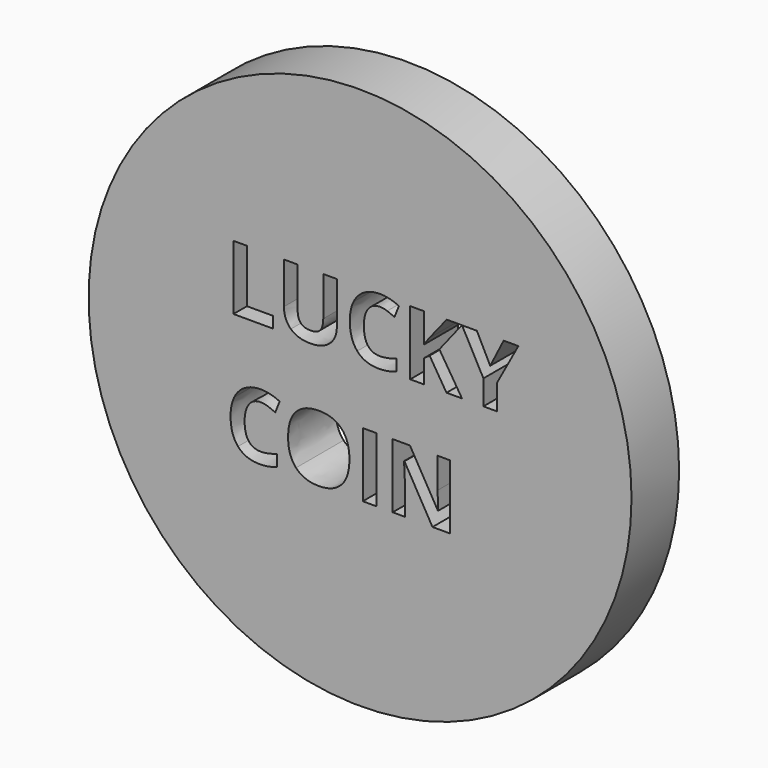
from build123d import *

# Parameters (mm, degrees)
F0_R     = 57.932951026
F0_W     = 2.9168109343
F0_H     = 13.753260226
F1_DEPTH = 12.7


with BuildPart() as f1:
    # F0 (on Front) → F1 (new body)
    with BuildSketch(Plane.XZ):
        Circle(F0_R)
        with BuildLine():
            add(Edge.make_bspline(
                [(-19.6506091277, -8.0144570558), (-20.4302314517, -7.7420407611), (-21.1827626525, -7.7420407611)],
                knots=[0, 0, 0, 1, 1, 1], degree=2))
            add(Edge.make_bspline(
                [(-21.1827626525, -7.7420407611), (-22.8293009199, -7.7420407611), (-23.7323383609, -8.9792020552)],
                knots=[0, 0, 0, 1, 1, 1], degree=2))
            add(Edge.make_bspline(
                [(-23.7323383609, -8.9792020552), (-24.6353758019, -10.2163633494), (-24.6353758019, -12.425794955)],
                knots=[0, 0, 0, 1, 1, 1], degree=2))
            add(Edge.make_bspline(
                [(-24.6353758019, -12.425794955), (-24.6353758019, -17.0252656543), (-21.1827626525, -17.0252656543)],
                knots=[0, 0, 0, 1, 1, 1], degree=2))
            add(Edge.make_bspline(
                [(-21.1827626525, -17.0252656543), (-19.7348926222, -17.0252656543), (-17.6759672568, -16.3028357015)],
                knots=[0, 0, 0, 1, 1, 1], degree=2))
            Line((-17.6759672568, -16.3028357015), (-17.6759672568, -18.7470570418))
            add(Edge.make_bspline(
                [(-17.6759672568, -18.7470570418), (-19.3676573962, -19.4544363705), (-21.4566840096, -19.4544363705)],
                knots=[0, 0, 0, 1, 1, 1], degree=2))
            add(Edge.make_bspline(
                [(-21.4566840096, -19.4544363705), (-24.4577784385, -19.4544363705), (-26.0471243346, -17.6333108646)],
                knots=[0, 0, 0, 1, 1, 1], degree=2))
            add(Edge.make_bspline(
                [(-26.0471243346, -17.6333108646), (-27.6364702307, -15.8121853586), (-27.6364702307, -12.4077342061)],
                knots=[0, 0, 0, 1, 1, 1], degree=2))
            add(Edge.make_bspline(
                [(-27.6364702307, -12.4077342061), (-27.6364702307, -10.2615152214), (-26.8553428443, -8.6480883269)],
                knots=[0, 0, 0, 1, 1, 1], degree=2))
            add(Edge.make_bspline(
                [(-26.8553428443, -8.6480883269), (-26.0742154578, -7.0346614323), (-24.6112948034, -6.175270801)],
                knots=[0, 0, 0, 1, 1, 1], degree=2))
            add(Edge.make_bspline(
                [(-24.6112948034, -6.175270801), (-23.1483741491, -5.3158801697), (-21.1827626525, -5.3158801697)],
                knots=[0, 0, 0, 1, 1, 1], degree=2))
            add(Edge.make_bspline(
                [(-21.1827626525, -5.3158801697), (-19.1810296584, -5.3158801697), (-17.1582257906, -6.2821302315)],
                knots=[0, 0, 0, 1, 1, 1], degree=2))
            Line((-17.1582257906, -6.2821302315), (-18.0973847292, -8.6541085765))
            add(Edge.make_bspline(
                [(-18.0973847292, -8.6541085765), (-18.8709868037, -8.2868733505), (-19.6506091277, -8.0144570558)],
                knots=[0, 0, 0, 1, 1, 1], degree=2))
        make_face(mode=Mode.SUBTRACT)
        with BuildLine():
            add(Edge.make_bspline(
                [(-3.9467880292, -7.1204499892), (-2.267138389, -8.9460906824), (-2.267138389, -12.3686025837)],
                knots=[0, 0, 0, 1, 1, 1], degree=2))
            add(Edge.make_bspline(
                [(-2.267138389, -12.3686025837), (-2.267138389, -15.7850942354), (-3.9603335908, -17.619765303)],
                knots=[0, 0, 0, 1, 1, 1], degree=2))
            add(Edge.make_bspline(
                [(-3.9603335908, -17.619765303), (-5.6535287926, -19.4544363705), (-8.814159836, -19.4544363705)],
                knots=[0, 0, 0, 1, 1, 1], degree=2))
            add(Edge.make_bspline(
                [(-8.814159836, -19.4544363705), (-11.9747908794, -19.4544363705), (-13.6679860812, -17.619765303)],
                knots=[0, 0, 0, 1, 1, 1], degree=2))
            add(Edge.make_bspline(
                [(-13.6679860812, -17.619765303), (-15.3611812831, -15.7850942354), (-15.3611812831, -12.3505418349)],
                knots=[0, 0, 0, 1, 1, 1], degree=2))
            add(Edge.make_bspline(
                [(-15.3611812831, -12.3505418349), (-15.3611812831, -8.9159894344), (-13.663470894, -7.1053993652)],
                knots=[0, 0, 0, 1, 1, 1], degree=2))
            add(Edge.make_bspline(
                [(-13.663470894, -7.1053993652), (-11.965760505, -5.2948092961), (-8.7960990872, -5.2948092961)],
                knots=[0, 0, 0, 1, 1, 1], degree=2))
            add(Edge.make_bspline(
                [(-8.7960990872, -5.2948092961), (-5.6264376694, -5.2948092961), (-3.9467880292, -7.1204499892)],
                knots=[0, 0, 0, 1, 1, 1], degree=2))
        make_face(mode=Mode.SUBTRACT)
        with Locations((2.0418552669, -12.3881683949)):
            Rectangle(F0_W, F0_H, mode=Mode.SUBTRACT)
        with BuildLine():
            Line((19.1619400853, -5.5115382819), (19.1619400853, -19.2647985079))
            Line((19.1619400853, -19.2647985079), (15.4564764525, -19.2647985079))
            Line((15.4564764525, -19.2647985079), (9.4723483437, -8.8618071879))
            Line((9.4723483437, -8.8618071879), (9.3880648492, -8.8618071879))
            add(Edge.make_bspline(
                [(9.3880648492, -8.8618071879), (9.5686723374, -11.6160713829), (9.5686723374, -12.793030181)],
                knots=[0, 0, 0, 1, 1, 1], degree=2))
            Line((9.5686723374, -12.793030181), (9.5686723374, -19.2647985079))
            Line((9.5686723374, -19.2647985079), (6.9619042578, -19.2647985079))
            Line((6.9619042578, -19.2647985079), (6.9619042578, -5.5115382819))
            Line((6.9619042578, -5.5115382819), (10.6402767673, -5.5115382819))
            Line((10.6402767673, -5.5115382819), (16.612364377, -15.8121853586))
            Line((16.612364377, -15.8121853586), (16.6785871226, -15.8121853586))
            add(Edge.make_bspline(
                [(16.6785871226, -15.8121853586), (16.5371112569, -13.1301641589), (16.5371112569, -12.0224382313)],
                knots=[0, 0, 0, 1, 1, 1], degree=2))
            Line((16.5371112569, -12.0224382313), (16.5371112569, -5.5115382819))
            Line((16.5371112569, -5.5115382819), (19.1619400853, -5.5115382819))
        make_face(mode=Mode.SUBTRACT)
        Polygon((-18.5308427009, 6.9353277795), (-27.0254148956, 6.9353277795), (-27.0254148956, 20.6885880055), (-24.1086039613, 20.6885880055), (-24.1086039613, 9.3434276221), (-18.5308427009, 9.3434276221), align=None, mode=Mode.SUBTRACT)
        with BuildLine():
            Line((-7.8539300238, 20.6885880055), (-4.9461494639, 20.6885880055))
            Line((-4.9461494639, 20.6885880055), (-4.9461494639, 11.7906590871))
            add(Edge.make_bspline(
                [(-4.9461494639, 11.7906590871), (-4.9461494639, 10.2645258119), (-5.6279427318, 9.1176682619)],
                knots=[0, 0, 0, 1, 1, 1], degree=2))
            add(Edge.make_bspline(
                [(-5.6279427318, 9.1176682619), (-6.3097359997, 7.9708107118), (-7.5995744779, 7.3582503144)],
                knots=[0, 0, 0, 1, 1, 1], degree=2))
            add(Edge.make_bspline(
                [(-7.5995744779, 7.3582503144), (-8.8894129561, 6.7456899169), (-10.6473258412, 6.7456899169)],
                knots=[0, 0, 0, 1, 1, 1], degree=2))
            add(Edge.make_bspline(
                [(-10.6473258412, 6.7456899169), (-13.2992457928, 6.7456899169), (-14.7666816344, 8.106266328)],
                knots=[0, 0, 0, 1, 1, 1], degree=2))
            add(Edge.make_bspline(
                [(-14.7666816344, 8.106266328), (-16.234117476, 9.466842739), (-16.234117476, 11.8267805848)],
                knots=[0, 0, 0, 1, 1, 1], degree=2))
            Line((-16.234117476, 11.8267805848), (-16.234117476, 20.6885880055))
            Line((-16.234117476, 20.6885880055), (-13.3293470409, 20.6885880055))
            Line((-13.3293470409, 20.6885880055), (-13.3293470409, 12.2692689308))
            add(Edge.make_bspline(
                [(-13.3293470409, 12.2692689308), (-13.3293470409, 10.6799230347), (-12.6896955202, 9.9364222083)],
                knots=[0, 0, 0, 1, 1, 1], degree=2))
            add(Edge.make_bspline(
                [(-12.6896955202, 9.9364222083), (-12.0500439995, 9.1929213819), (-10.5720727211, 9.1929213819)],
                knots=[0, 0, 0, 1, 1, 1], degree=2))
            add(Edge.make_bspline(
                [(-10.5720727211, 9.1929213819), (-9.1422634396, 9.1929213819), (-8.4980967317, 9.9409373955)],
                knots=[0, 0, 0, 1, 1, 1], degree=2))
            add(Edge.make_bspline(
                [(-8.4980967317, 9.9409373955), (-7.8539300238, 10.6889534091), (-7.8539300238, 12.2873296797)],
                knots=[0, 0, 0, 1, 1, 1], degree=2))
            Line((-7.8539300238, 12.2873296797), (-7.8539300238, 20.6885880055))
        make_face(mode=Mode.SUBTRACT)
        with BuildLine():
            add(Edge.make_bspline(
                [(5.7969859589, 18.1856692316), (5.0173636349, 18.4580855263), (4.2648324341, 18.4580855263)],
                knots=[0, 0, 0, 1, 1, 1], degree=2))
            add(Edge.make_bspline(
                [(4.2648324341, 18.4580855263), (2.6182941667, 18.4580855263), (1.7152567257, 17.2209242322)],
                knots=[0, 0, 0, 1, 1, 1], degree=2))
            add(Edge.make_bspline(
                [(1.7152567257, 17.2209242322), (0.8122192848, 15.983762938), (0.8122192848, 13.7743313325)],
                knots=[0, 0, 0, 1, 1, 1], degree=2))
            add(Edge.make_bspline(
                [(0.8122192848, 13.7743313325), (0.8122192848, 9.1748606331), (4.2648324341, 9.1748606331)],
                knots=[0, 0, 0, 1, 1, 1], degree=2))
            add(Edge.make_bspline(
                [(4.2648324341, 9.1748606331), (5.7127024644, 9.1748606331), (7.7716278298, 9.8972905859)],
                knots=[0, 0, 0, 1, 1, 1], degree=2))
            Line((7.7716278298, 9.8972905859), (7.7716278298, 7.4530692457))
            add(Edge.make_bspline(
                [(7.7716278298, 7.4530692457), (6.0799376904, 6.7456899169), (3.990911077, 6.7456899169)],
                knots=[0, 0, 0, 1, 1, 1], degree=2))
            add(Edge.make_bspline(
                [(3.990911077, 6.7456899169), (0.9898166481, 6.7456899169), (-0.599529248, 8.5668154229)],
                knots=[0, 0, 0, 1, 1, 1], degree=2))
            add(Edge.make_bspline(
                [(-0.599529248, 8.5668154229), (-2.1888751441, 10.3879409288), (-2.1888751441, 13.7923920813)],
                knots=[0, 0, 0, 1, 1, 1], degree=2))
            add(Edge.make_bspline(
                [(-2.1888751441, 13.7923920813), (-2.1888751441, 15.938611066), (-1.4077477576, 17.5520379605)],
                knots=[0, 0, 0, 1, 1, 1], degree=2))
            add(Edge.make_bspline(
                [(-1.4077477576, 17.5520379605), (-0.6266203712, 19.1654648551), (0.8363002832, 20.0248554864)],
                knots=[0, 0, 0, 1, 1, 1], degree=2))
            add(Edge.make_bspline(
                [(0.8363002832, 20.0248554864), (2.2992209376, 20.8842461177), (4.2648324341, 20.8842461177)],
                knots=[0, 0, 0, 1, 1, 1], degree=2))
            add(Edge.make_bspline(
                [(4.2648324341, 20.8842461177), (6.2665654282, 20.8842461177), (8.289369296, 19.9179960559)],
                knots=[0, 0, 0, 1, 1, 1], degree=2))
            Line((8.289369296, 19.9179960559), (7.3502103574, 17.5460177109))
            add(Edge.make_bspline(
                [(7.3502103574, 17.5460177109), (6.576608283, 17.9132529369), (5.7969859589, 18.1856692316)],
                knots=[0, 0, 0, 1, 1, 1], degree=2))
        make_face(mode=Mode.SUBTRACT)
        Polygon((16.9254173565, 14.6021156534), (21.7596777905, 6.9353277795), (18.448540507, 6.9353277795), (14.8454211175, 12.7298180257), (13.6142800729, 11.8448413336), (13.6142800729, 6.9353277795), (10.6974691386, 6.9353277795), (10.6974691386, 20.6885880055), (13.6142800729, 20.6885880055), (13.6142800729, 14.3944170419), (14.761137623, 16.0138641861), (18.4876721294, 20.6885880055), (21.7235562929, 20.6885880055), align=None, mode=Mode.SUBTRACT)
        Polygon((24.9203088339, 20.6885880055), (27.7708970226, 15.0265432506), (30.6395459601, 20.6885880055), (33.7821162547, 20.6885880055), (29.218767053, 12.2873296797), (29.218767053, 6.9353277795), (26.3230269922, 6.9353277795), (26.3230269922, 12.1940158108), (21.7596777905, 20.6885880055), align=None, mode=Mode.SUBTRACT)
    extrude(amount=F1_DEPTH)


solid = f1.part
